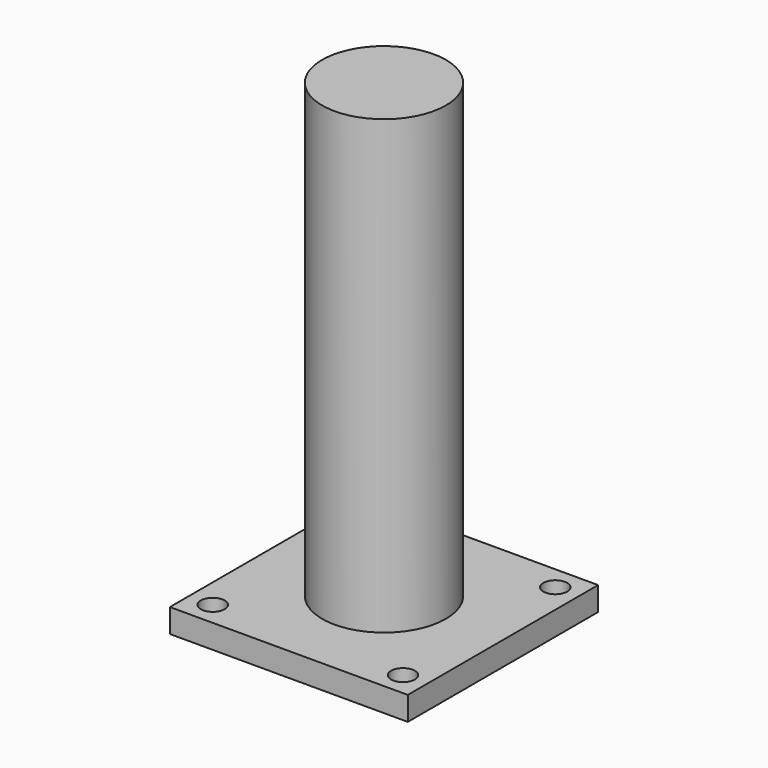
from build123d import *

# Parameters (mm, degrees)
F0_R     = 13
F1_DEPTH = 100
F2_W     = 50
F2_H     = 50
F2_R     = 2.5
F3_DEPTH = 5
F4_R     = 17.5
F4_R_2   = 13
F5_DEPTH = 5


# Not quite as in the source:
# - a fillet or chamfer that OpenCascade refuses, or shapes differently, is made with other operations: its cross-section is extruded or revolved along the edge and cut away or added


with BuildPart() as f1:
    # F0 (on Top) → F1 (new body)
    with BuildSketch(Plane.XY):
        Circle(F0_R)
    extrude(amount=F1_DEPTH)


with BuildPart() as f3:
    # F2 (on Top) → F3 (new body)
    with BuildSketch(Plane.XY):
        Rectangle(F2_W, F2_H)
        with Locations((-20, -20)):
            Circle(F2_R, mode=Mode.SUBTRACT)
        with Locations((20, -20)):
            Circle(F2_R, mode=Mode.SUBTRACT)
        with Locations((-20, 20)):
            Circle(F2_R, mode=Mode.SUBTRACT)
        with Locations((20, 20)):
            Circle(F2_R, mode=Mode.SUBTRACT)
    extrude(amount=F3_DEPTH)


with BuildPart() as f5:
    # F4 (on Top) → F5 (new body)
    with BuildSketch(Plane.XY):
        Circle(F4_R)
        Circle(F4_R_2, mode=Mode.SUBTRACT)
    extrude(amount=F5_DEPTH)

    # F6: chamfer of 5 on 1 edges, made by hand

    # F6_s1 → F6_t2 (revolve, cut)
    with BuildSketch(Plane.XZ):
        Polygon((17.5, 0), (12.5, 5), (17.5, 5), align=None)
    revolve(axis=Axis((0, 0, 5), (0, 0, 1)), mode=Mode.SUBTRACT)


solid = Compound([f1.part, f3.part, f5.part])
